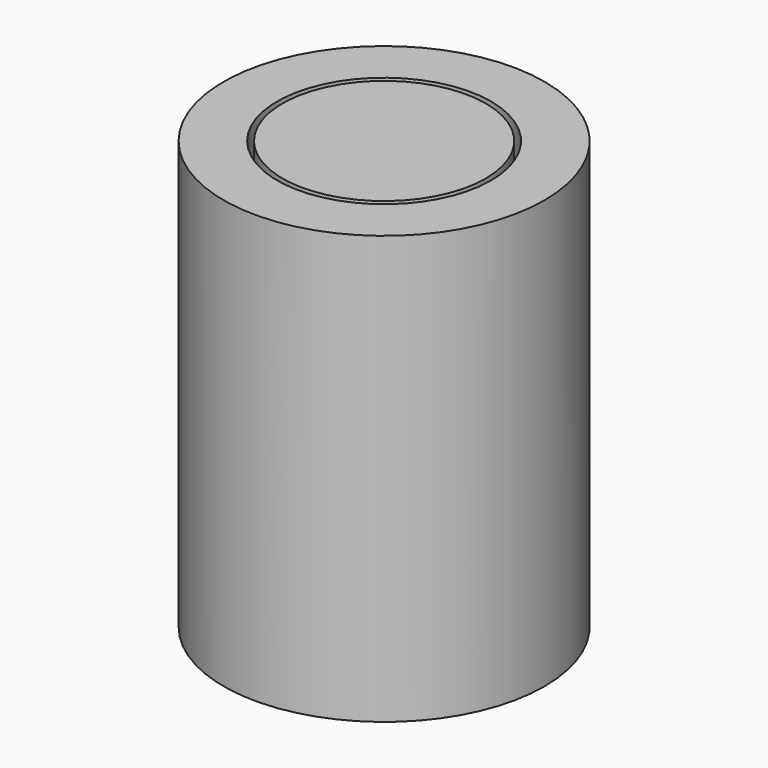
from build123d import *

# Parameters (mm, degrees)
F0_R     = 7.5
F0_R_2   = 5
F1_DEPTH = 20
F2_R     = 4.75
F3_DEPTH = 20


# Not quite as in the source:
# - a feature names something its author has since deleted; it is built from what else it names


with BuildPart() as f1:
    # F0 (on Top) → F1 (new body)
    with BuildSketch(Plane.XY):
        with Locations((54.9561347067, 55.4606581624)):
            Circle(F0_R)
        with Locations((54.9561347067, 55.4606581624)):
            Circle(F0_R_2, mode=Mode.SUBTRACT)
    extrude(amount=F1_DEPTH)


with BuildPart() as f3:
    # F2 (on Top) → F3 (new body)
    with BuildSketch(Plane.XY):
        with Locations((54.9561347067, 55.4606581624)):
            Circle(F2_R)
    extrude(amount=F3_DEPTH)


solid = Compound([f1.part, f3.part])
